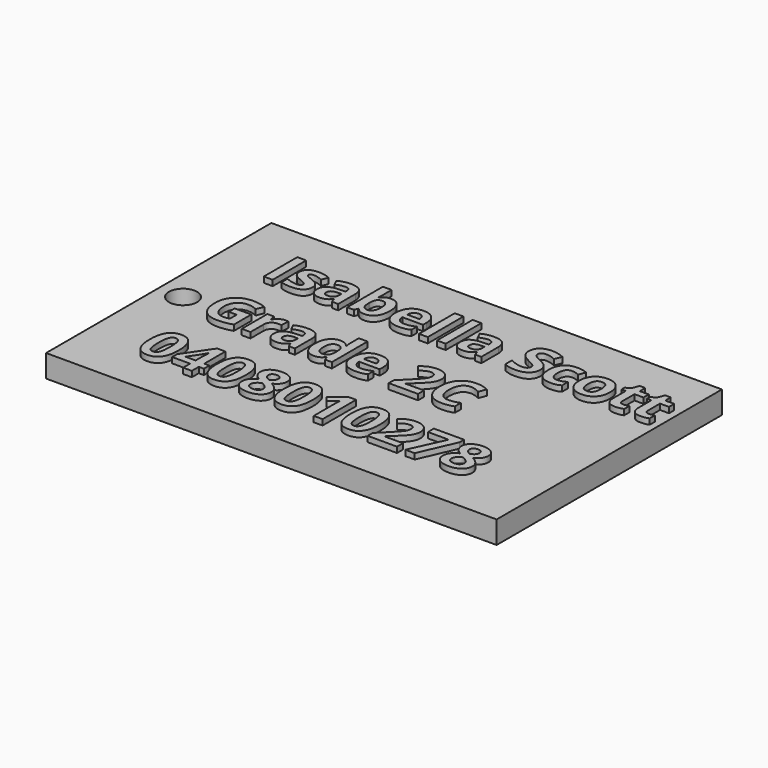
from build123d import *

# Parameters (mm, degrees)
F0_W         = 80
F0_H         = 50
F0_R         = 2.5
F1_DEPTH     = 4
F2_TEXT_SIZE = 10.4244229337
F4_DEPTH     = 5
F5_DEPTH     = 5


# Not quite as in the source:
# - Text() gives the source's letters only with a copy of the font that has no kerning and outlines rounded to 1/6400 em; it was checked with that copy


with BuildPart() as f1:
    # F0 (on Top) → F1 (new body)
    with BuildSketch(Plane.XY):
        with Locations((-0.5432310091, -25)):
            Rectangle(F0_W, F0_H)
        with Locations((-36.2217649817, -25.0000003725)):
            Circle(F0_R, mode=Mode.SUBTRACT)
    extrude(amount=-F1_DEPTH)


with BuildPart() as f1_1:
    # F3: moved
    add(f1.part.moved(Location((0, 0, -1))))

    # F2 (on face) → F4 (cut)
    with BuildSketch(Plane.XY):
        with Locations((-31.0586265661, -14.7059382871)):
            Text('Isabella Scott', F2_TEXT_SIZE, font='Open Sans', font_style=FontStyle.BOLD, text_align=(TextAlign.LEFT, TextAlign.BOTTOM))
        with Locations((-31.0586265661, -28.883153477)):
            Text('Grade 2C', F2_TEXT_SIZE, font='Open Sans', font_style=FontStyle.BOLD, text_align=(TextAlign.LEFT, TextAlign.BOTTOM))
        with Locations((-31.0586265661, -43.0603686668)):
            Text('0408010278', F2_TEXT_SIZE, font='Open Sans', font_style=FontStyle.BOLD, text_align=(TextAlign.LEFT, TextAlign.BOTTOM))
    extrude(amount=-F4_DEPTH, mode=Mode.SUBTRACT)


with BuildPart() as f5:
    # F2 (on face) → F5 (new body)
    with BuildSketch(Plane.XY):
        with Locations((-31.0586265661, -14.7059382871)):
            Text('Isabella Scott', F2_TEXT_SIZE, font='Open Sans', font_style=FontStyle.BOLD, text_align=(TextAlign.LEFT, TextAlign.BOTTOM))
        with Locations((-31.0586265661, -28.883153477)):
            Text('Grade 2C', F2_TEXT_SIZE, font='Open Sans', font_style=FontStyle.BOLD, text_align=(TextAlign.LEFT, TextAlign.BOTTOM))
        with Locations((-31.0586265661, -43.0603686668)):
            Text('0408010278', F2_TEXT_SIZE, font='Open Sans', font_style=FontStyle.BOLD, text_align=(TextAlign.LEFT, TextAlign.BOTTOM))
    extrude(amount=-F5_DEPTH)


solid = Compound([f1_1.part, f5.part])
